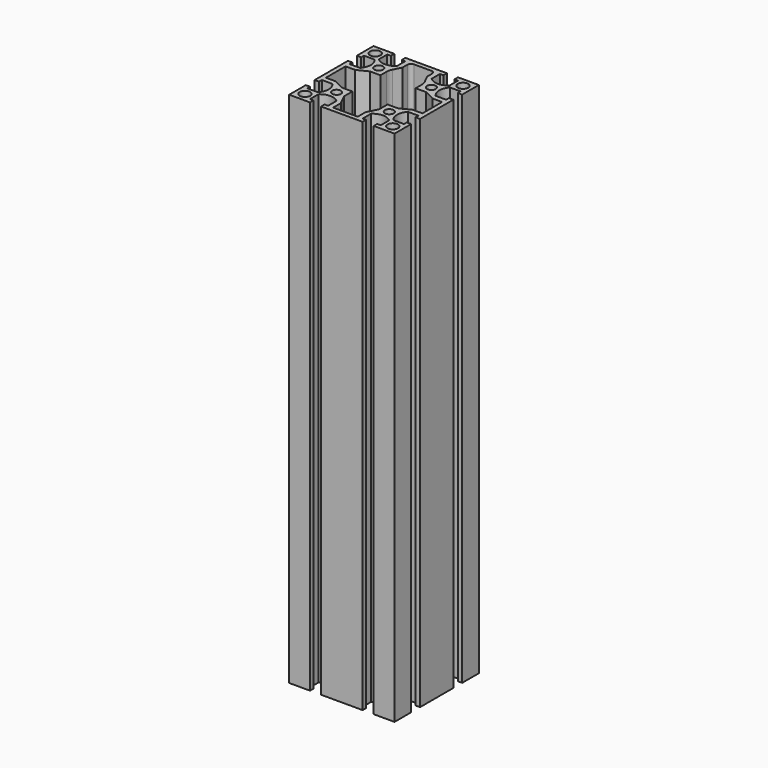
from build123d import *

# Parameters (mm, degrees)
F0_R     = 3
F0_R_2   = 2.5
F1_DEPTH = 295
F2_R     = 2
F3_R     = 7


# Not quite as in the source:
# - a feature names something its author has since deleted; it is built from what else it names


with BuildPart() as f1:
    # F0 (on Top) → F1 (new body)
    with BuildSketch(Plane.XY):
        with BuildLine():
            Line((18.15, -30), (30, -30))
            Line((30, -30), (30, -18.15))
            Line((30, -18.15), (27.5, -18.15))
            Line((27.5, -18.15), (27.5, -20.15))
            Line((27.5, -20.15), (21.5477069044, -20.15))
            ThreePointArc((21.5477069044, -20.15), (19.5, -15), (21.5477069044, -9.85))
            Line((21.5477069044, -9.85), (27.5, -9.85))
            Line((27.5, -9.85), (27.5, -11.85))
            Line((27.5, -11.85), (30, -11.85))
            Line((30, -11.85), (30, 11.85))
            Line((30, 11.85), (27.5, 11.85))
            Line((27.5, 11.85), (27.5, 9.85))
            Line((27.5, 9.85), (21.5477069044, 9.85))
            ThreePointArc((21.5477069044, 9.85), (19.5, 15), (21.5477069044, 20.15))
            Line((21.5477069044, 20.15), (27.5, 20.15))
            Line((27.5, 20.15), (27.5, 18.15))
            Line((27.5, 18.15), (30, 18.15))
            Line((30, 18.15), (30, 30))
            Line((30, 30), (18.15, 30))
            Line((18.15, 30), (18.15, 27.5))
            Line((18.15, 27.5), (20.15, 27.5))
            Line((20.15, 27.5), (20.15, 21.5477069044))
            ThreePointArc((20.15, 21.5477069044), (15, 19.5), (9.85, 21.5477069044))
            Line((9.85, 21.5477069044), (9.85, 27.5))
            Line((9.85, 27.5), (11.85, 27.5))
            Line((11.85, 27.5), (11.85, 30))
            Line((11.85, 30), (-11.85, 30))
            Line((-11.85, 30), (-11.85, 27.5))
            Line((-11.85, 27.5), (-9.85, 27.5))
            Line((-9.85, 27.5), (-9.85, 21.5477069044))
            ThreePointArc((-9.85, 21.5477069044), (-15, 19.5), (-20.15, 21.5477069044))
            Line((-20.15, 21.5477069044), (-20.15, 27.5))
            Line((-20.15, 27.5), (-18.15, 27.5))
            Line((-18.15, 27.5), (-18.15, 30))
            Line((-18.15, 30), (-30, 30))
            Line((-30, 30), (-30, 18.15))
            Line((-30, 18.15), (-27.5, 18.15))
            Line((-27.5, 18.15), (-27.5, 20.15))
            Line((-27.5, 20.15), (-21.5477069044, 20.15))
            ThreePointArc((-21.5477069044, 20.15), (-19.5, 15), (-21.5477069044, 9.85))
            Line((-21.5477069044, 9.85), (-27.5, 9.85))
            Line((-27.5, 9.85), (-27.5, 11.85))
            Line((-27.5, 11.85), (-30, 11.85))
            Line((-30, 11.85), (-30, -11.85))
            Line((-30, -11.85), (-27.5, -11.85))
            Line((-27.5, -11.85), (-27.5, -9.85))
            Line((-27.5, -9.85), (-21.5477069044, -9.85))
            ThreePointArc((-21.5477069044, -9.85), (-19.5, -15), (-21.5477069044, -20.15))
            Line((-21.5477069044, -20.15), (-27.5, -20.15))
            Line((-27.5, -20.15), (-27.5, -18.15))
            Line((-27.5, -18.15), (-30, -18.15))
            Line((-30, -18.15), (-30, -30))
            Line((-30, -30), (-18.15, -30))
            Line((-18.15, -30), (-18.15, -27.5))
            Line((-18.15, -27.5), (-20.15, -27.5))
            Line((-20.15, -27.5), (-20.15, -21.5477069044))
            ThreePointArc((-20.15, -21.5477069044), (-15, -19.5), (-9.85, -21.5477069044))
            Line((-9.85, -21.5477069044), (-9.85, -27.5))
            Line((-9.85, -27.5), (-11.85, -27.5))
            Line((-11.85, -27.5), (-11.85, -30))
            Line((-11.85, -30), (11.85, -30))
            Line((11.85, -30), (11.85, -27.5))
            Line((11.85, -27.5), (9.85, -27.5))
            Line((9.85, -27.5), (9.85, -21.5477069044))
            ThreePointArc((9.85, -21.5477069044), (15, -19.5), (20.15, -21.5477069044))
            Line((20.15, -21.5477069044), (20.15, -27.5))
            Line((20.15, -27.5), (18.15, -27.5))
            Line((18.15, -27.5), (18.15, -30))
        make_face()
        with Locations((-25, -25)):
            Circle(F0_R, mode=Mode.SUBTRACT)
        with Locations((-15, -15)):
            Circle(F0_R_2, mode=Mode.SUBTRACT)
        with Locations((25, -25)):
            Circle(F0_R, mode=Mode.SUBTRACT)
        with Locations((15, -15)):
            Circle(F0_R_2, mode=Mode.SUBTRACT)
        with Locations((-25, 25)):
            Circle(F0_R, mode=Mode.SUBTRACT)
        with Locations((-15, 15)):
            Circle(F0_R_2, mode=Mode.SUBTRACT)
        Polygon((-7, 22), (-7, 27.5), (0, 27.5), (7, 27.5), (7, 22), (10, 16), (10, 10), (16, 10), (22, 7), (27.5, 7), (27.5, 0), (27.5, -7), (22, -7), (16, -10), (10, -10), (10, -16), (7, -22), (7, -27.5), (0, -27.5), (-7, -27.5), (-7, -22), (-10, -16), (-10, -10), (-16, -10), (-22, -7), (-27.5, -7), (-27.5, 0), (-27.5, 7), (-22, 7), (-16, 10), (-10, 10), (-10, 16), align=None, mode=Mode.SUBTRACT)
        with Locations((15, 15)):
            Circle(F0_R_2, mode=Mode.SUBTRACT)
        with Locations((25, 25)):
            Circle(F0_R, mode=Mode.SUBTRACT)
    extrude(amount=F1_DEPTH)

    # F2
    f2_edges = [f1.edges().sort_by_distance(p)[0] for p in [
        (-7, 27.5, 147.5),
        (7, 27.5, 147.5),
    ]]
    fillet(f2_edges, radius=F2_R)

    # F3
    f3_edges = [f1.edges().sort_by_distance(p)[0] for p in [
        (-10, 16, 147.5),
        (10, 16, 147.5),
    ]]
    fillet(f3_edges, radius=F3_R)


solid = f1.part
